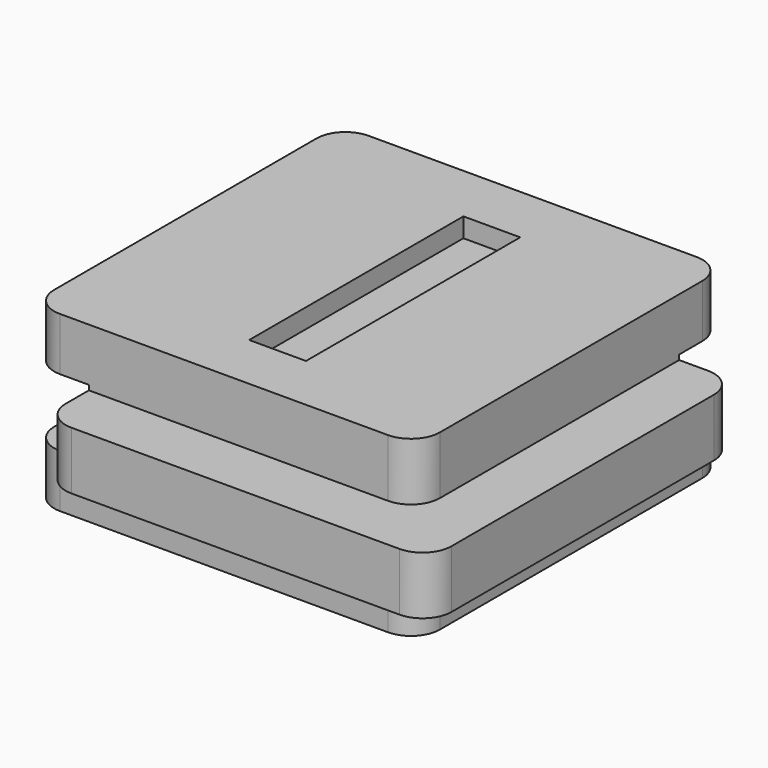
from build123d import *

# Parameters (mm, degrees)
F0_W         = 14
F0_H         = 3
F0_W_2       = 3
F1_DEPTH     = 20
F2_DEPTH     = 3
F3_W         = 3
F3_H         = 3
F4_DEPTH     = 100
F5_W         = 3
F5_H         = 3.5
F6_DEPTH     = 100
F7_R         = 1.5
F8_TEXT_SIZE = 19.4444444444
F9_DEPTH     = 1


# Not quite as in the source:
# - Text() gives the source's letters only with a copy of the font that has no kerning and outlines rounded to 1/6400 em; it was checked with that copy


with BuildPart() as f1:
    # F0 (on Front) → F1 (new body)
    with BuildSketch(Plane.XZ):
        Polygon((10, 1.5), (10, 4.5), (-10, 4.5), (-10, 1.5), (-7, 1.5), (7, 1.5), align=None)
        Rectangle(F0_W, F0_H)
        with Locations((11.5, 0)):
            Rectangle(F0_W_2, F0_H)
        with Locations((8.5, 0)):
            Rectangle(F0_W_2, F0_H)
        with Locations((-8.5, 0)):
            Rectangle(F0_W_2, F0_H)
        Polygon((10, -4.5), (10, -1.5), (7, -1.5), (-7, -1.5), (-10, -1.5), (-10, -4.5), align=None)
    extrude(amount=-F1_DEPTH)

    # F0 (on Front) → F2 (join)
    with BuildSketch(Plane.XZ):
        with Locations((-8.5, 0)):
            Rectangle(F0_W_2, F0_H)
        Rectangle(F0_W, F0_H)
        with Locations((8.5, 0)):
            Rectangle(F0_W_2, F0_H)
        with Locations((11.5, 0)):
            Rectangle(F0_W_2, F0_H)
    extrude(amount=F2_DEPTH)

    # F3 (on face) → F4 (cut)
    with BuildSketch(Plane.YZ.offset(13)):
        Polygon((23, -1.75), (23, 1.75), (17, 1.75), (17, 1.5), (20, 1.5), (20, -1.5), (17, -1.5), (17, -1.75), align=None)
        with Locations((18.5, 0)):
            Rectangle(F3_W, F3_H)
    extrude(amount=-F4_DEPTH, mode=Mode.SUBTRACT)

    # F5 (on face) → F6 (cut)
    with BuildSketch(Plane(origin=(0, 17, 0), x_dir=(-1, 0, 0), z_dir=(0, 1, 0))):
        with Locations((11.5, 0)):
            Rectangle(F5_W, F5_H)
        with Locations((8.5, 0)):
            Rectangle(F5_W, F5_H)
    extrude(amount=-F6_DEPTH, mode=Mode.SUBTRACT)

    # F7
    f7_edges = [f1.edges().sort_by_distance(p)[0] for p in [
        (-7, -3, 0),
        (13, -3, 0),
        (10, 0, 3),
        (10, 0, -3),
        (-10, 0, -3.125),
        (-10, 0, 3.125),
        (-7, 17, 0),
        (-10, 20, 3.125),
        (-10, 20, -3.125),
        (13, 17, 0),
        (10, 20, 3.125),
        (10, 20, -3.125),
    ]]
    fillet(f7_edges, radius=F7_R)

    # F8 (on face) → F9 (cut)
    with BuildSketch(Plane.XY.offset(4.5)):
        with Locations((-2.8348682146, 3)):
            Text('I', F8_TEXT_SIZE, font='Open Sans', font_style=FontStyle.BOLD, text_align=(TextAlign.LEFT, TextAlign.BOTTOM))
    extrude(amount=-F9_DEPTH, mode=Mode.SUBTRACT)


solid = f1.part
